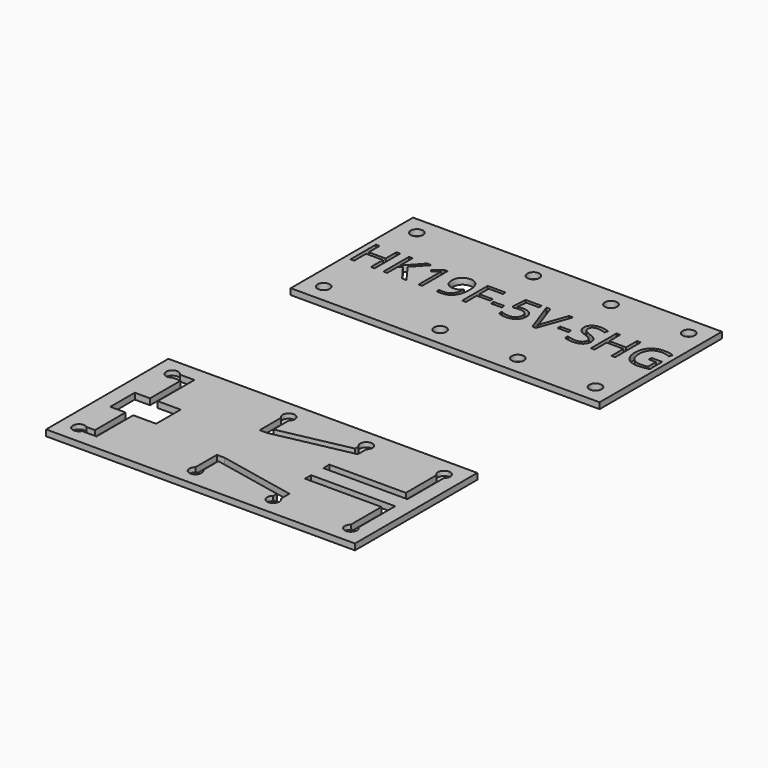
from build123d import *
from build123d import SkipClean  # not in build123d's __all__

# Parameters (mm, degrees)
F0_W     = 20.2
F0_H     = 10
F0_R     = 0.4
F0_W_2   = 0.7020916289
F0_H_2   = 0.2174012541
F1_DEPTH = 0.4
F2_DEPTH = 0.4
F3_DEPTH = 0.1
F4_DEPTH = 0.4


with BuildPart() as f1:
    # F0 (on Top) → F1 (new body)
    with BuildSketch(Plane.XY):
        Rectangle(F0_W, F0_H)
        with Locations((-8.9, -3.81)):
            Circle(F0_R, mode=Mode.SUBTRACT)
        with Locations((-1.28, -3.81)):
            Circle(F0_R, mode=Mode.SUBTRACT)
        Polygon((-8.1248569729, 1.4821502128), (-8.1248569729, -0.6090210078), (-8.3678886906, -0.6090210078), (-8.3678886906, 0.3750057211), (-9.4695409401, 0.3750057211), (-9.4695409401, -0.6090210078), (-9.7125726578, -0.6090210078), (-9.7125726578, 1.4821502128), (-9.4695409401, 1.4821502128), (-9.4695409401, 0.5924069751), (-8.3678886906, 0.5924069751), (-8.3678886906, 1.4821502128), align=None, mode=Mode.SUBTRACT)
        Polygon((-6.9133598792, 0.5736418143), (-6.0410087418, -0.6090210078), (-6.3270630235, -0.6090210078), (-7.0891116298, 0.4052130532), (-7.3083436313, 0.2106961417), (-7.3083436313, -0.6090210078), (-7.551375349, -0.6090210078), (-7.551375349, 1.4821502128), (-7.3083436313, 1.4821502128), (-7.3083436313, 0.4450318092), (-6.3600164767, 1.4821502128), (-6.0725891345, 1.4821502128), align=None, mode=Mode.SUBTRACT)
        with BuildLine():
            Line((-5.0185363175, 1.4821502128), (-5.0185363175, -0.6090210078))
            Line((-5.0185363175, -0.6090210078), (-5.2501258639, -0.6090210078))
            Line((-5.2501258639, -0.6090210078), (-5.2501258639, 0.8812073779))
            add(Edge.make_bspline(
                [(-5.2501258639, 0.8812073779), (-5.2501258639, 1.0674859261), (-5.2386836926, 1.2331685661)],
                knots=[0, 0, 0, 1, 1, 1], degree=2))
            add(Edge.make_bspline(
                [(-5.2386836926, 1.2331685661), (-5.2684333379, 1.2029612339), (-5.3057348162, 1.1702366241)],
                knots=[0, 0, 0, 1, 1, 1], degree=2))
            add(Edge.make_bspline(
                [(-5.3057348162, 1.1702366241), (-5.3430362946, 1.1375120143), (-5.6460249897, 0.8912764886)],
                knots=[0, 0, 0, 1, 1, 1], degree=2))
            Line((-5.6460249897, 0.8912764886), (-5.7718888736, 1.0542130075))
            Line((-5.7718888736, 1.0542130075), (-5.2185454712, 1.4821502128))
            Line((-5.2185454712, 1.4821502128), (-5.0185363175, 1.4821502128))
        make_face(mode=Mode.SUBTRACT)
        with Locations((-8.9, 3.81)):
            Circle(F0_R, mode=Mode.SUBTRACT)
        with BuildLine():
            add(Edge.make_bspline(
                [(-2.934459243, 1.0837338093), (-2.8486429585, 0.8743420752), (-2.8486429585, 0.589660854)],
                knots=[0, 0, 0, 1, 1, 1], degree=2))
            add(Edge.make_bspline(
                [(-2.8486429585, 0.589660854), (-2.8486429585, -0.6378552794), (-3.7983431736, -0.6378552794)],
                knots=[0, 0, 0, 1, 1, 1], degree=2))
            add(Edge.make_bspline(
                [(-3.7983431736, -0.6378552794), (-3.9644835004, -0.6378552794), (-4.0615131127, -0.6090210078)],
                knots=[0, 0, 0, 1, 1, 1], degree=2))
            Line((-4.0615131127, -0.6090210078), (-4.0615131127, -0.4044349856))
            add(Edge.make_bspline(
                [(-4.0615131127, -0.4044349856), (-3.9470914001, -0.4415076205), (-3.8015469816, -0.4415076205)],
                knots=[0, 0, 0, 1, 1, 1], degree=2))
            add(Edge.make_bspline(
                [(-3.8015469816, -0.4415076205), (-3.4582818436, -0.4415076205), (-3.2829877798, -0.2291409218)],
                knots=[0, 0, 0, 1, 1, 1], degree=2))
            add(Edge.make_bspline(
                [(-3.2829877798, -0.2291409218), (-3.107693716, -0.0167742231), (-3.092132363, 0.4221474667)],
                knots=[0, 0, 0, 1, 1, 1], degree=2))
            Line((-3.092132363, 0.4221474667), (-3.1090667765, 0.4221474667))
            add(Edge.make_bspline(
                [(-3.1090667765, 0.4221474667), (-3.1877889148, 0.3036065724), (-3.3180008238, 0.2413611607)],
                knots=[0, 0, 0, 1, 1, 1], degree=2))
            add(Edge.make_bspline(
                [(-3.3180008238, 0.2413611607), (-3.4482127328, 0.179115749), (-3.6111492517, 0.179115749)],
                knots=[0, 0, 0, 1, 1, 1], degree=2))
            add(Edge.make_bspline(
                [(-3.6111492517, 0.179115749), (-3.8885074832, 0.179115749), (-4.0516728454, 0.3450272324)],
                knots=[0, 0, 0, 1, 1, 1], degree=2))
            add(Edge.make_bspline(
                [(-4.0516728454, 0.3450272324), (-4.2148382077, 0.5109387157), (-4.2148382077, 0.8084351687)],
                knots=[0, 0, 0, 1, 1, 1], degree=2))
            add(Edge.make_bspline(
                [(-4.2148382077, 0.8084351687), (-4.2148382077, 1.1343082063), (-4.0324499977, 1.3231040322)],
                knots=[0, 0, 0, 1, 1, 1], degree=2))
            add(Edge.make_bspline(
                [(-4.0324499977, 1.3231040322), (-3.8500617877, 1.5118998581), (-3.5525653348, 1.5118998581)],
                knots=[0, 0, 0, 1, 1, 1], degree=2))
            add(Edge.make_bspline(
                [(-3.5525653348, 1.5118998581), (-3.3392832624, 1.5118998581), (-3.1797793949, 1.4025127008)],
                knots=[0, 0, 0, 1, 1, 1], degree=2))
            add(Edge.make_bspline(
                [(-3.1797793949, 1.4025127008), (-3.0202755275, 1.2931255435), (-2.934459243, 1.0837338093)],
                knots=[0, 0, 0, 1, 1, 1], degree=2))
        make_face(mode=Mode.SUBTRACT)
        Polygon((-2.1611973088, 0.2848414115), (-2.1611973088, -0.6090210078), (-2.4042290265, -0.6090210078), (-2.4042290265, 1.4821502128), (-1.2385006179, 1.4821502128), (-1.2385006179, 1.2661220193), (-2.1611973088, 1.2661220193), (-2.1611973088, 0.500869605), (-1.2943384137, 0.500869605), (-1.2943384137, 0.2848414115), align=None, mode=Mode.SUBTRACT)
        with Locations((-0.7084992448, 0.1761407845)):
            Rectangle(F0_W_2, F0_H_2, mode=Mode.SUBTRACT)
        with Locations((-1.28, 3.81)):
            Circle(F0_R, mode=Mode.SUBTRACT)
        with Locations((3.8, -3.81)):
            Circle(F0_R, mode=Mode.SUBTRACT)
        with Locations((8.88, -3.81)):
            Circle(F0_R, mode=Mode.SUBTRACT)
        with BuildLine():
            add(Edge.make_bspline(
                [(0.2315895464, 0.6354295391), (0.3958991258, 0.6683829924), (0.5592933315, 0.6683829924)],
                knots=[0, 0, 0, 1, 1, 1], degree=2))
            add(Edge.make_bspline(
                [(0.5592933315, 0.6683829924), (0.8897432377, 0.6683829924), (1.0792255938, 0.5045310998)],
                knots=[0, 0, 0, 1, 1, 1], degree=2))
            add(Edge.make_bspline(
                [(1.0792255938, 0.5045310998), (1.26870795, 0.3406792073), (1.26870795, 0.0559979862)],
                knots=[0, 0, 0, 1, 1, 1], degree=2))
            add(Edge.make_bspline(
                [(1.26870795, 0.0559979862), (1.26870795, -0.2685019909), (1.0620623369, -0.4531786352)],
                knots=[0, 0, 0, 1, 1, 1], degree=2))
            add(Edge.make_bspline(
                [(1.0620623369, -0.4531786352), (0.8554167239, -0.6378552794), (0.4920133645, -0.6378552794)],
                knots=[0, 0, 0, 1, 1, 1], degree=2))
            add(Edge.make_bspline(
                [(0.4920133645, -0.6378552794), (0.1386791157, -0.6378552794), (-0.0471417456, -0.5248066273)],
                knots=[0, 0, 0, 1, 1, 1], degree=2))
            Line((-0.0471417456, -0.5248066273), (-0.0471417456, -0.295963202))
            add(Edge.make_bspline(
                [(-0.0471417456, -0.295963202), (0.0526339878, -0.3600393611), (0.2013822143, -0.3966543091)],
                knots=[0, 0, 0, 1, 1, 1], degree=2))
            add(Edge.make_bspline(
                [(0.2013822143, -0.3966543091), (0.3501304408, -0.4332692572), (0.4947594856, -0.4332692572)],
                knots=[0, 0, 0, 1, 1, 1], degree=2))
            add(Edge.make_bspline(
                [(0.4947594856, -0.4332692572), (0.7464872534, -0.4332692572), (0.8858528994, -0.3144995194)],
                knots=[0, 0, 0, 1, 1, 1], degree=2))
            add(Edge.make_bspline(
                [(0.8858528994, -0.3144995194), (1.0252185455, -0.1957297817), (1.0252185455, 0.028994462)],
                knots=[0, 0, 0, 1, 1, 1], degree=2))
            add(Edge.make_bspline(
                [(1.0252185455, 0.028994462), (1.0252185455, 0.4665430912), (0.4892672434, 0.4665430912)],
                knots=[0, 0, 0, 1, 1, 1], degree=2))
            add(Edge.make_bspline(
                [(0.4892672434, 0.4665430912), (0.3533342487, 0.4665430912), (0.1258638839, 0.4248935878)],
                knots=[0, 0, 0, 1, 1, 1], degree=2))
            Line((0.1258638839, 0.4248935878), (0.0027461211, 0.5036157261))
            Line((0.0027461211, 0.5036157261), (0.0814682594, 1.4821502128))
            Line((0.0814682594, 1.4821502128), (1.1213327841, 1.4821502128))
            Line((1.1213327841, 1.4821502128), (1.1213327841, 1.2633758982))
            Line((1.1213327841, 1.2633758982), (0.2846812211, 1.2633758982))
            Line((0.2846812211, 1.2633758982), (0.2315895464, 0.6354295391))
        make_face(mode=Mode.SUBTRACT)
        with BuildLine():
            Line((2.4413016614, 0.1374662456), (2.9191267335, 1.4821502128))
            Line((2.9191267335, 1.4821502128), (3.1804659252, 1.4821502128))
            Line((3.1804659252, 1.4821502128), (2.427113369, -0.6090210078))
            Line((2.427113369, -0.6090210078), (2.1868277724, -0.6090210078))
            Line((2.1868277724, -0.6090210078), (1.4371367111, 1.4821502128))
            Line((1.4371367111, 1.4821502128), (1.694814408, 1.4821502128))
            Line((1.694814408, 1.4821502128), (2.1753856012, 0.1292278823))
            add(Edge.make_bspline(
                [(2.1753856012, 0.1292278823), (2.2582269211, -0.1041924116), (2.3067417273, -0.3243397867)],
                knots=[0, 0, 0, 1, 1, 1], degree=2))
            add(Edge.make_bspline(
                [(2.3067417273, -0.3243397867), (2.3584603414, -0.0927502403), (2.4413016614, 0.1374662456)],
                knots=[0, 0, 0, 1, 1, 1], degree=2))
        make_face(mode=Mode.SUBTRACT)
        with Locations((3.6518833814, 0.1761407845)):
            Rectangle(F0_W_2, F0_H_2, mode=Mode.SUBTRACT)
        with BuildLine():
            add(Edge.make_bspline(
                [(5.4666117442, 0.2962835828), (5.5901871939, 0.1617236487), (5.5901871939, -0.0524737974)],
                knots=[0, 0, 0, 1, 1, 1], degree=2))
            add(Edge.make_bspline(
                [(5.5901871939, -0.0524737974), (5.5901871939, -0.3284589684), (5.3899491968, -0.4831571239)],
                knots=[0, 0, 0, 1, 1, 1], degree=2))
            add(Edge.make_bspline(
                [(5.3899491968, -0.4831571239), (5.1897111996, -0.6378552794), (4.8464460616, -0.6378552794)],
                knots=[0, 0, 0, 1, 1, 1], degree=2))
            add(Edge.make_bspline(
                [(4.8464460616, -0.6378552794), (4.4748043389, -0.6378552794), (4.2743374983, -0.5417410408)],
                knots=[0, 0, 0, 1, 1, 1], degree=2))
            Line((4.2743374983, -0.5417410408), (4.2743374983, -0.3074053732))
            add(Edge.make_bspline(
                [(4.2743374983, -0.3074053732), (4.4034051902, -0.3614124216), (4.5548995377, -0.3929928143)],
                knots=[0, 0, 0, 1, 1, 1], degree=2))
            add(Edge.make_bspline(
                [(4.5548995377, -0.3929928143), (4.7063938853, -0.424573207), (4.8551421118, -0.424573207)],
                knots=[0, 0, 0, 1, 1, 1], degree=2))
            add(Edge.make_bspline(
                [(4.8551421118, -0.424573207), (5.0981738295, -0.424573207), (5.2212915923, -0.3323493066)],
                knots=[0, 0, 0, 1, 1, 1], degree=2))
            add(Edge.make_bspline(
                [(5.2212915923, -0.3323493066), (5.3444093551, -0.2401254062), (5.3444093551, -0.07535814)],
                knots=[0, 0, 0, 1, 1, 1], degree=2))
            add(Edge.make_bspline(
                [(5.3444093551, -0.07535814), (5.3444093551, 0.0331136436), (5.3007002609, 0.1024532015)],
                knots=[0, 0, 0, 1, 1, 1], degree=2))
            add(Edge.make_bspline(
                [(5.3007002609, 0.1024532015), (5.2569911666, 0.1717927594), (5.1546981555, 0.2306055197)],
                knots=[0, 0, 0, 1, 1, 1], degree=2))
            add(Edge.make_bspline(
                [(5.1546981555, 0.2306055197), (5.0524051444, 0.28941828), (4.8436999405, 0.3635635498)],
                knots=[0, 0, 0, 1, 1, 1], degree=2))
            add(Edge.make_bspline(
                [(4.8436999405, 0.3635635498), (4.5521534166, 0.4679161518), (4.426976063, 0.6109432926)],
                knots=[0, 0, 0, 1, 1, 1], degree=2))
            add(Edge.make_bspline(
                [(4.426976063, 0.6109432926), (4.3017987093, 0.7539704334), (4.3017987093, 0.9841869193)],
                knots=[0, 0, 0, 1, 1, 1], degree=2))
            add(Edge.make_bspline(
                [(4.3017987093, 0.9841869193), (4.3017987093, 1.2258455765), (4.4832715456, 1.3688727173)],
                knots=[0, 0, 0, 1, 1, 1], degree=2))
            add(Edge.make_bspline(
                [(4.4832715456, 1.3688727173), (4.6647443819, 1.5118998581), (4.9640715822, 1.5118998581)],
                knots=[0, 0, 0, 1, 1, 1], degree=2))
            add(Edge.make_bspline(
                [(4.9640715822, 1.5118998581), (5.2757563275, 1.5118998581), (5.5375532061, 1.3974781455)],
                knots=[0, 0, 0, 1, 1, 1], degree=2))
            Line((5.5375532061, 1.3974781455), (5.4615771889, 1.1860268204))
            add(Edge.make_bspline(
                [(5.4615771889, 1.1860268204), (5.2025264314, 1.2944986041), (4.9581216532, 1.2944986041)],
                knots=[0, 0, 0, 1, 1, 1], degree=2))
            add(Edge.make_bspline(
                [(4.9581216532, 1.2944986041), (4.7649778022, 1.2944986041), (4.6562771752, 1.2116572841)],
                knots=[0, 0, 0, 1, 1, 1], degree=2))
            add(Edge.make_bspline(
                [(4.6562771752, 1.2116572841), (4.5475765481, 1.1288159641), (4.5475765481, 0.9814407982)],
                knots=[0, 0, 0, 1, 1, 1], degree=2))
            add(Edge.make_bspline(
                [(4.5475765481, 0.9814407982), (4.5475765481, 0.8729690146), (4.5876241476, 0.8034006133)],
                knots=[0, 0, 0, 1, 1, 1], degree=2))
            add(Edge.make_bspline(
                [(4.5876241476, 0.8034006133), (4.627671747, 0.733832212), (4.7228706119, 0.6759348254)],
                knots=[0, 0, 0, 1, 1, 1], degree=2))
            add(Edge.make_bspline(
                [(4.7228706119, 0.6759348254), (4.8180694769, 0.6180374388), (5.0139594489, 0.5480113506)],
                knots=[0, 0, 0, 1, 1, 1], degree=2))
            add(Edge.make_bspline(
                [(5.0139594489, 0.5480113506), (5.3430362946, 0.4308435169), (5.4666117442, 0.2962835828)],
                knots=[0, 0, 0, 1, 1, 1], degree=2))
        make_face(mode=Mode.SUBTRACT)
        with Locations((3.8, 3.81)):
            Circle(F0_R, mode=Mode.SUBTRACT)
        Polygon((7.6058400842, 1.4821502128), (7.6058400842, -0.6090210078), (7.3628083665, -0.6090210078), (7.3628083665, 0.3750057211), (6.261156117, 0.3750057211), (6.261156117, -0.6090210078), (6.0181243993, -0.6090210078), (6.0181243993, 1.4821502128), (6.261156117, 1.4821502128), (6.261156117, 0.5924069751), (7.3628083665, 0.5924069751), (7.3628083665, 1.4821502128), align=None, mode=Mode.SUBTRACT)
        with BuildLine():
            Line((9.0992722779, 0.2692800586), (9.0992722779, 0.4866813126))
            Line((9.0992722779, 0.4866813126), (9.810059957, 0.4866813126))
            Line((9.810059957, 0.4866813126), (9.810059957, -0.5302988695))
            add(Edge.make_bspline(
                [(9.810059957, -0.5302988695), (9.6439196302, -0.5833905442), (9.4722870612, -0.6106229118)],
                knots=[0, 0, 0, 1, 1, 1], degree=2))
            add(Edge.make_bspline(
                [(9.4722870612, -0.6106229118), (9.3006544922, -0.6378552794), (9.074557188, -0.6378552794)],
                knots=[0, 0, 0, 1, 1, 1], degree=2))
            add(Edge.make_bspline(
                [(9.074557188, -0.6378552794), (8.5999359238, -0.6378552794), (8.3353929242, -0.3552336491)],
                knots=[0, 0, 0, 1, 1, 1], degree=2))
            add(Edge.make_bspline(
                [(8.3353929242, -0.3552336491), (8.0708499245, -0.0726120189), (8.0708499245, 0.4363357591)],
                knots=[0, 0, 0, 1, 1, 1], degree=2))
            add(Edge.make_bspline(
                [(8.0708499245, 0.4363357591), (8.0708499245, 0.7626664836), (8.2017483638, 1.0079866355)],
                knots=[0, 0, 0, 1, 1, 1], degree=2))
            add(Edge.make_bspline(
                [(8.2017483638, 1.0079866355), (8.3326468031, 1.2533067875), (8.5786534853, 1.3826033228)],
                knots=[0, 0, 0, 1, 1, 1], degree=2))
            add(Edge.make_bspline(
                [(8.5786534853, 1.3826033228), (8.8246601675, 1.5118998581), (9.1546523868, 1.5118998581)],
                knots=[0, 0, 0, 1, 1, 1], degree=2))
            add(Edge.make_bspline(
                [(9.1546523868, 1.5118998581), (9.4896791615, 1.5118998581), (9.7784795643, 1.3892397821)],
                knots=[0, 0, 0, 1, 1, 1], degree=2))
            Line((9.7784795643, 1.3892397821), (9.684196073, 1.1745846492))
            add(Edge.make_bspline(
                [(9.684196073, 1.1745846492), (9.4008879125, 1.2944986041), (9.1390910339, 1.2944986041)],
                knots=[0, 0, 0, 1, 1, 1], degree=2))
            add(Edge.make_bspline(
                [(9.1390910339, 1.2944986041), (8.7573802005, 1.2944986041), (8.5427250675, 1.0672570827)],
                knots=[0, 0, 0, 1, 1, 1], degree=2))
            add(Edge.make_bspline(
                [(8.5427250675, 1.0672570827), (8.3280699346, 0.8400155614), (8.3280699346, 0.4363357591)],
                knots=[0, 0, 0, 1, 1, 1], degree=2))
            add(Edge.make_bspline(
                [(8.3280699346, 0.4363357591), (8.3280699346, 0.0129754222), (8.5347155476, -0.2057988924)],
                knots=[0, 0, 0, 1, 1, 1], degree=2))
            add(Edge.make_bspline(
                [(8.5347155476, -0.2057988924), (8.7413611607, -0.424573207), (9.141837155, -0.424573207)],
                knots=[0, 0, 0, 1, 1, 1], degree=2))
            add(Edge.make_bspline(
                [(9.141837155, -0.424573207), (9.3592384091, -0.424573207), (9.5665705524, -0.3742276534)],
                knots=[0, 0, 0, 1, 1, 1], degree=2))
            Line((9.5665705524, -0.3742276534), (9.5665705524, 0.2692800586))
            Line((9.5665705524, 0.2692800586), (9.0992722779, 0.2692800586))
        make_face(mode=Mode.SUBTRACT)
        with Locations((8.88, 3.81)):
            Circle(F0_R, mode=Mode.SUBTRACT)
    extrude(amount=F1_DEPTH)


with BuildPart() as f2:
    # F0 (on Top) → F2 (new body)
    with BuildSketch(Plane.XY):
        with Locations((0, -20)):
            Rectangle(F0_W, F0_H)
        with BuildLine():
            Line((-8.1, -16.5), (-8.6472155068, -16.5))
            ThreePointArc((-8.6472155068, -16.5), (-9.2923510579, -16.1121498405), (-8.5480056819, -16))
            Line((-8.5480056819, -16), (-8.1, -16))
            Line((-8.1, -16), (-7.6, -16))
            Line((-7.6, -16), (-7.6, -19))
            Line((-7.6, -19), (-6.1, -19))
            Line((-6.1, -19), (-6.1, -21))
            Line((-6.1, -21), (-7.6, -21))
            Line((-7.6, -21), (-7.6, -24))
            Line((-7.6, -24), (-8.1, -24))
            Line((-8.1, -24), (-8.5480056819, -24))
            ThreePointArc((-8.5480056819, -24), (-9.2923510579, -23.8878501595), (-8.6472155068, -23.5))
            Line((-8.6472155068, -23.5), (-8.1, -23.5))
            Line((-8.1, -23.5), (-8.1, -21))
            Line((-8.1, -21), (-9.1, -21))
            Line((-9.1, -21), (-9.1, -19))
            Line((-9.1, -19), (-8.1, -19))
            Line((-8.1, -19), (-8.1, -16.5))
        make_face(mode=Mode.SUBTRACT)
        with BuildLine():
            ThreePointArc((-1.03, -23.4977501001), (-0.9194448725, -23.6367949192), (-0.88, -23.81))
            ThreePointArc((-0.88, -23.81), (-1.4532050808, -24.1705551275), (-1.53, -23.4977501001))
            Line((-1.53, -23.4977501001), (-1.53, -21.7477501001))
            Line((-1.53, -21.7477501001), (-1.03, -21.7477501001))
            Line((-1.03, -21.7477501001), (4.05, -22.7977501001))
            Line((4.05, -22.7977501001), (4.05, -23.1977501001))
            Line((4.05, -23.1977501001), (4.05, -23.4977501001))
            ThreePointArc((4.05, -23.4977501001), (4.1605551275, -23.6367949192), (4.2, -23.81))
            ThreePointArc((4.2, -23.81), (3.6267949192, -24.1705551275), (3.55, -23.4977501001))
            Line((3.55, -23.4977501001), (3.55, -23.1977501001))
            Line((3.55, -23.1977501001), (-1.03, -22.2477501001))
            Line((-1.03, -22.2477501001), (-1.03, -23.4977501001))
        make_face(mode=Mode.SUBTRACT)
        with BuildLine():
            ThreePointArc((9.13, -23.4977501001), (9.2405551275, -23.6367949192), (9.28, -23.81))
            ThreePointArc((9.28, -23.81), (8.7067949192, -24.1705551275), (8.63, -23.4977501001))
            Line((8.63, -23.4977501001), (8.63, -20.9977501001))
            Line((8.63, -20.9977501001), (3.63, -20.9977501001))
            Line((3.63, -20.9977501001), (3.63, -20.4977501001))
            Line((3.63, -20.4977501001), (9.13, -20.4977501001))
            Line((9.13, -20.4977501001), (9.13, -20.9977501001))
            Line((9.13, -20.9977501001), (9.13, -23.4977501001))
        make_face(mode=Mode.SUBTRACT)
        with BuildLine():
            ThreePointArc((8.63, -16.5022498999), (8.7067949192, -15.8294448725), (9.28, -16.19))
            ThreePointArc((9.28, -16.19), (9.2405551275, -16.3632050808), (9.13, -16.5022498999))
            Line((9.13, -16.5022498999), (9.13, -19.0022498999))
            Line((9.13, -19.0022498999), (9.13, -19.5022498999))
            Line((9.13, -19.5022498999), (3.63, -19.5022498999))
            Line((3.63, -19.5022498999), (3.63, -19.0022498999))
            Line((3.63, -19.0022498999), (8.63, -19.0022498999))
            Line((8.63, -19.0022498999), (8.63, -16.5022498999))
        make_face(mode=Mode.SUBTRACT)
        with BuildLine():
            ThreePointArc((-1.53, -16.5022498999), (-1.4532050808, -15.8294448725), (-0.88, -16.19))
            ThreePointArc((-0.88, -16.19), (-0.9194448725, -16.3632050808), (-1.03, -16.5022498999))
            Line((-1.03, -16.5022498999), (-1.03, -17.7522498999))
            Line((-1.03, -17.7522498999), (3.55, -16.8022498999))
            Line((3.55, -16.8022498999), (3.55, -16.5022498999))
            ThreePointArc((3.55, -16.5022498999), (3.6267949192, -15.8294448725), (4.2, -16.19))
            ThreePointArc((4.2, -16.19), (4.1605551275, -16.3632050808), (4.05, -16.5022498999))
            Line((4.05, -16.5022498999), (4.05, -16.8022498999))
            Line((4.05, -16.8022498999), (4.05, -17.2022498999))
            Line((4.05, -17.2022498999), (-1.03, -18.2522498999))
            Line((-1.03, -18.2522498999), (-1.53, -18.2522498999))
            Line((-1.53, -18.2522498999), (-1.53, -16.5022498999))
        make_face(mode=Mode.SUBTRACT)
    extrude(amount=F2_DEPTH)

    # F0 (on Top) → F3 (join)
    with BuildSketch(Plane.XY):
        with BuildLine():
            ThreePointArc((9.13, -16.5022498999), (9.2405551275, -16.3632050808), (9.28, -16.19))
            ThreePointArc((9.28, -16.19), (8.7067949192, -15.8294448725), (8.63, -16.5022498999))
            Line((8.63, -16.5022498999), (9.13, -16.5022498999))
        make_face()
        with BuildLine():
            Line((9.13, -16.5022498999), (8.63, -16.5022498999))
            ThreePointArc((8.63, -16.5022498999), (8.88, -16.59), (9.13, -16.5022498999))
        make_face()
        with BuildLine():
            ThreePointArc((4.2, -16.19), (3.6267949192, -15.8294448725), (3.55, -16.5022498999))
            Line((3.55, -16.5022498999), (4.05, -16.5022498999))
            ThreePointArc((4.05, -16.5022498999), (4.1605551275, -16.3632050808), (4.2, -16.19))
        make_face()
        with BuildLine():
            Line((4.05, -16.5022498999), (3.55, -16.5022498999))
            ThreePointArc((3.55, -16.5022498999), (3.8, -16.59), (4.05, -16.5022498999))
        make_face()
        with BuildLine():
            ThreePointArc((-1.03, -16.5022498999), (-0.9194448725, -16.3632050808), (-0.88, -16.19))
            ThreePointArc((-0.88, -16.19), (-1.4532050808, -15.8294448725), (-1.53, -16.5022498999))
            Line((-1.53, -16.5022498999), (-1.03, -16.5022498999))
        make_face()
        with BuildLine():
            Line((-1.03, -16.5022498999), (-1.53, -16.5022498999))
            ThreePointArc((-1.53, -16.5022498999), (-1.28, -16.59), (-1.03, -16.5022498999))
        make_face()
        with BuildLine():
            ThreePointArc((-8.5480056819, -16), (-9.2923510579, -16.1121498405), (-8.6472155068, -16.5))
            Line((-8.6472155068, -16.5), (-8.6472155068, -16))
            Line((-8.6472155068, -16), (-8.5480056819, -16))
        make_face()
        with BuildLine():
            Line((-8.6472155068, -16), (-8.6472155068, -16.5))
            ThreePointArc((-8.6472155068, -16.5), (-8.5386734183, -16.3615899221), (-8.5, -16.19))
            ThreePointArc((-8.5, -16.19), (-8.5121870765, -16.0920146114), (-8.5480056819, -16))
            Line((-8.5480056819, -16), (-8.6472155068, -16))
        make_face()
        with BuildLine():
            Line((-8.6472155068, -24), (-8.6472155068, -23.5))
            ThreePointArc((-8.6472155068, -23.5), (-9.2923510579, -23.8878501595), (-8.5480056819, -24))
            Line((-8.5480056819, -24), (-8.6472155068, -24))
        make_face()
        with BuildLine():
            ThreePointArc((-8.5, -23.81), (-8.5386734183, -23.6384100779), (-8.6472155068, -23.5))
            Line((-8.6472155068, -23.5), (-8.6472155068, -24))
            Line((-8.6472155068, -24), (-8.5480056819, -24))
            ThreePointArc((-8.5480056819, -24), (-8.5121870765, -23.9079853886), (-8.5, -23.81))
        make_face()
        with BuildLine():
            ThreePointArc((-1.53, -23.4977501001), (-1.4532050808, -24.1705551275), (-0.88, -23.81))
            ThreePointArc((-0.88, -23.81), (-0.9194448725, -23.6367949192), (-1.03, -23.4977501001))
            Line((-1.03, -23.4977501001), (-1.53, -23.4977501001))
        make_face()
        with BuildLine():
            Line((-1.53, -23.4977501001), (-1.03, -23.4977501001))
            ThreePointArc((-1.03, -23.4977501001), (-1.28, -23.41), (-1.53, -23.4977501001))
        make_face()
        with BuildLine():
            ThreePointArc((4.05, -23.4977501001), (3.8, -23.41), (3.55, -23.4977501001))
            Line((3.55, -23.4977501001), (4.05, -23.4977501001))
        make_face()
        with BuildLine():
            Line((4.05, -23.4977501001), (3.55, -23.4977501001))
            ThreePointArc((3.55, -23.4977501001), (3.6267949192, -24.1705551275), (4.2, -23.81))
            ThreePointArc((4.2, -23.81), (4.1605551275, -23.6367949192), (4.05, -23.4977501001))
        make_face()
        with BuildLine():
            Line((8.63, -23.4977501001), (9.13, -23.4977501001))
            ThreePointArc((9.13, -23.4977501001), (8.88, -23.41), (8.63, -23.4977501001))
        make_face()
        with BuildLine():
            ThreePointArc((8.63, -23.4977501001), (8.7067949192, -24.1705551275), (9.28, -23.81))
            ThreePointArc((9.28, -23.81), (9.2405551275, -23.6367949192), (9.13, -23.4977501001))
            Line((9.13, -23.4977501001), (8.63, -23.4977501001))
        make_face()
    extrude(amount=F3_DEPTH)

    # F0 (on Top) → F4 (join)
    with BuildSketch(Plane.XY):
        with BuildLine():
            Line((-8.6472155068, -24), (-8.6472155068, -23.5))
            ThreePointArc((-8.6472155068, -23.5), (-9.2923510579, -23.8878501595), (-8.5480056819, -24))
            Line((-8.5480056819, -24), (-8.6472155068, -24))
        make_face()
        with BuildLine():
            ThreePointArc((-8.5, -23.81), (-8.5386734183, -23.6384100779), (-8.6472155068, -23.5))
            Line((-8.6472155068, -23.5), (-8.6472155068, -24))
            Line((-8.6472155068, -24), (-8.5480056819, -24))
            ThreePointArc((-8.5480056819, -24), (-8.5121870765, -23.9079853886), (-8.5, -23.81))
        make_face()
        with BuildLine():
            ThreePointArc((-1.53, -23.4977501001), (-1.4532050808, -24.1705551275), (-0.88, -23.81))
            ThreePointArc((-0.88, -23.81), (-0.9194448725, -23.6367949192), (-1.03, -23.4977501001))
            Line((-1.03, -23.4977501001), (-1.53, -23.4977501001))
        make_face()
        with BuildLine():
            Line((-1.53, -23.4977501001), (-1.03, -23.4977501001))
            ThreePointArc((-1.03, -23.4977501001), (-1.28, -23.41), (-1.53, -23.4977501001))
        make_face()
        with BuildLine():
            Line((4.05, -23.4977501001), (3.55, -23.4977501001))
            ThreePointArc((3.55, -23.4977501001), (3.6267949192, -24.1705551275), (4.2, -23.81))
            ThreePointArc((4.2, -23.81), (4.1605551275, -23.6367949192), (4.05, -23.4977501001))
        make_face()
        with BuildLine():
            ThreePointArc((4.05, -23.4977501001), (3.8, -23.41), (3.55, -23.4977501001))
            Line((3.55, -23.4977501001), (4.05, -23.4977501001))
        make_face()
        with BuildLine():
            ThreePointArc((8.63, -23.4977501001), (8.7067949192, -24.1705551275), (9.28, -23.81))
            ThreePointArc((9.28, -23.81), (9.2405551275, -23.6367949192), (9.13, -23.4977501001))
            Line((9.13, -23.4977501001), (8.63, -23.4977501001))
        make_face()
        with BuildLine():
            Line((8.63, -23.4977501001), (9.13, -23.4977501001))
            ThreePointArc((9.13, -23.4977501001), (8.88, -23.41), (8.63, -23.4977501001))
        make_face()
        with BuildLine():
            Line((9.13, -16.5022498999), (8.63, -16.5022498999))
            ThreePointArc((8.63, -16.5022498999), (8.88, -16.59), (9.13, -16.5022498999))
        make_face()
        with BuildLine():
            ThreePointArc((9.13, -16.5022498999), (9.2405551275, -16.3632050808), (9.28, -16.19))
            ThreePointArc((9.28, -16.19), (8.7067949192, -15.8294448725), (8.63, -16.5022498999))
            Line((8.63, -16.5022498999), (9.13, -16.5022498999))
        make_face()
        with BuildLine():
            Line((4.05, -16.5022498999), (3.55, -16.5022498999))
            ThreePointArc((3.55, -16.5022498999), (3.8, -16.59), (4.05, -16.5022498999))
        make_face()
        with BuildLine():
            ThreePointArc((4.2, -16.19), (3.6267949192, -15.8294448725), (3.55, -16.5022498999))
            Line((3.55, -16.5022498999), (4.05, -16.5022498999))
            ThreePointArc((4.05, -16.5022498999), (4.1605551275, -16.3632050808), (4.2, -16.19))
        make_face()
        with BuildLine():
            Line((-1.03, -16.5022498999), (-1.53, -16.5022498999))
            ThreePointArc((-1.53, -16.5022498999), (-1.28, -16.59), (-1.03, -16.5022498999))
        make_face()
        with BuildLine():
            ThreePointArc((-1.03, -16.5022498999), (-0.9194448725, -16.3632050808), (-0.88, -16.19))
            ThreePointArc((-0.88, -16.19), (-1.4532050808, -15.8294448725), (-1.53, -16.5022498999))
            Line((-1.53, -16.5022498999), (-1.03, -16.5022498999))
        make_face()
        with BuildLine():
            Line((-8.6472155068, -16), (-8.6472155068, -16.5))
            ThreePointArc((-8.6472155068, -16.5), (-8.5386734183, -16.3615899221), (-8.5, -16.19))
            ThreePointArc((-8.5, -16.19), (-8.5121870765, -16.0920146114), (-8.5480056819, -16))
            Line((-8.5480056819, -16), (-8.6472155068, -16))
        make_face()
        with BuildLine():
            ThreePointArc((-8.5480056819, -16), (-9.2923510579, -16.1121498405), (-8.6472155068, -16.5))
            Line((-8.6472155068, -16.5), (-8.6472155068, -16))
            Line((-8.6472155068, -16), (-8.5480056819, -16))
        make_face()
    with SkipClean():  # cleaning this boolean's faces spoils the solid; the shape is the same uncleaned
        extrude(amount=-F4_DEPTH)


solid = Compound([f1.part, f2.part])
